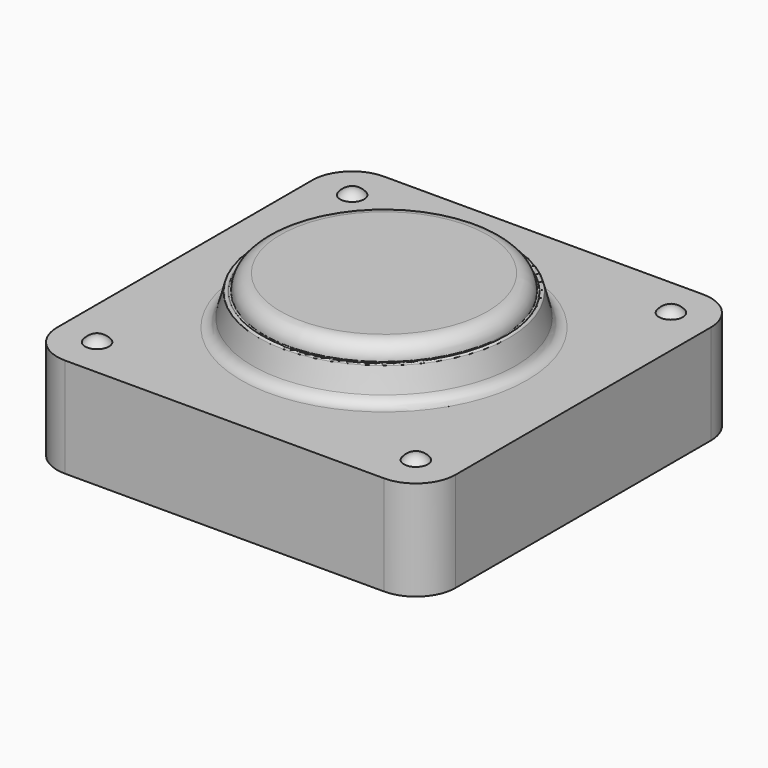
from build123d import *

# Parameters (mm, degrees)
F1_DEPTH        = 25
F6_COPIES_COUNT = 4


# Not quite as in the source:
# - a pattern or mirror of a feature is missing from the dataset's text; its kind, count and spacing are read off the source's solid


with BuildPart() as f1:
    # F0 (on Top) → F1 (new body)
    with BuildSketch(Plane.XY):
        with BuildLine():
            ThreePointArc((50, 40), (47.0710678119, 47.0710678119), (40, 50))
            Line((40, 50), (-40, 50))
            ThreePointArc((-40, 50), (-47.0710678119, 47.0710678119), (-50, 40))
            Line((-50, 40), (-50, -40))
            ThreePointArc((-50, -40), (-47.0710678119, -47.0710678119), (-40, -50))
            Line((-40, -50), (40, -50))
            ThreePointArc((40, -50), (47.0710678119, -47.0710678119), (50, -40))
            Line((50, -40), (50, 40))
        make_face()
    extrude(amount=F1_DEPTH)

    # F2 (on Front) → F3 (revolve)
    with BuildSketch(Plane.XZ):
        with BuildLine():
            Line((26, 37), (0, 37))
            Line((0, 37), (0, 25))
            Line((0, 25), (35.8856441977, 25))
            ThreePointArc((35.8856441977, 25), (34.0593599107, 25.6199399791), (32.9878667188, 27.2235428647))
            Line((32.9878667188, 27.2235428647), (31.4574072829, 32.9352952387))
            ThreePointArc((31.4574072829, 32.9352952387), (30.9744443697, 33.3058857162), (30.4914814566, 32.9352952387))
            ThreePointArc((30.4914814566, 32.9352952387), (30.2173684519, 32.7521387847), (30, 33))
            ThreePointArc((30, 33), (28.8284271247, 35.8284271247), (26, 37))
        make_face()
    revolve(axis=Axis((0, 0, 32.0425145328), (0, 0, 1)))

    # F5 (on plane+point) → F6 (revolve)
    with BuildSketch(Plane.XZ.offset(40)):
        with BuildLine():
            Line((-40, 26.5), (-40, 25))
            Line((-40, 25), (-37, 25))
            ThreePointArc((-37, 25), (-38.3229490169, 26.1041019662), (-40, 26.5))
        make_face()
    f6 = revolve(axis=Axis((-40, -40, 31.9980286476), (0, 0, 1)))

    # F6_copies: F6 ×4 about axis
    f6_copies_axis = Axis((0, 0, 0), (0, 0, 1))
    for i in range(1, F6_COPIES_COUNT):
        add(f6.rotate(f6_copies_axis, i * 360 / F6_COPIES_COUNT))


solid = f1.part
